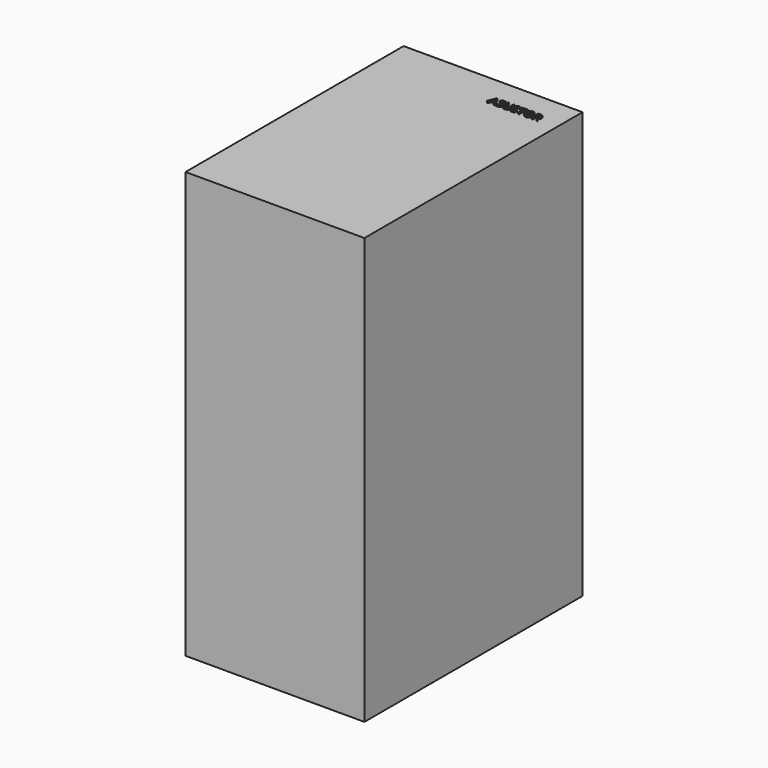
from build123d import *

# Parameters (mm, degrees)
F0_W         = 105
F0_H         = 160
F1_DEPTH     = 250
F2_TEXT_SIZE = 6.7316457471
F3_DEPTH     = 1


# Not quite as in the source:
# - Text() gives the source's letters only with a copy of the font that has no kerning and outlines rounded to 1/6400 em; it was checked with that copy


with BuildPart() as f1:
    # F0 (on Top) → F1 (new body)
    with BuildSketch(Plane.XY):
        with Locations((-52.5, 80)):
            Rectangle(F0_W, F0_H)
    extrude(amount=F1_DEPTH)

    # F2 (on face) → F3 (join)
    with BuildSketch(Plane.XY.offset(250)):
        with Locations((-40, 140)):
            Text('ASUSTOR', F2_TEXT_SIZE, font='Open Sans', text_align=(TextAlign.LEFT, TextAlign.BOTTOM))
    extrude(amount=F3_DEPTH)


solid = f1.part
